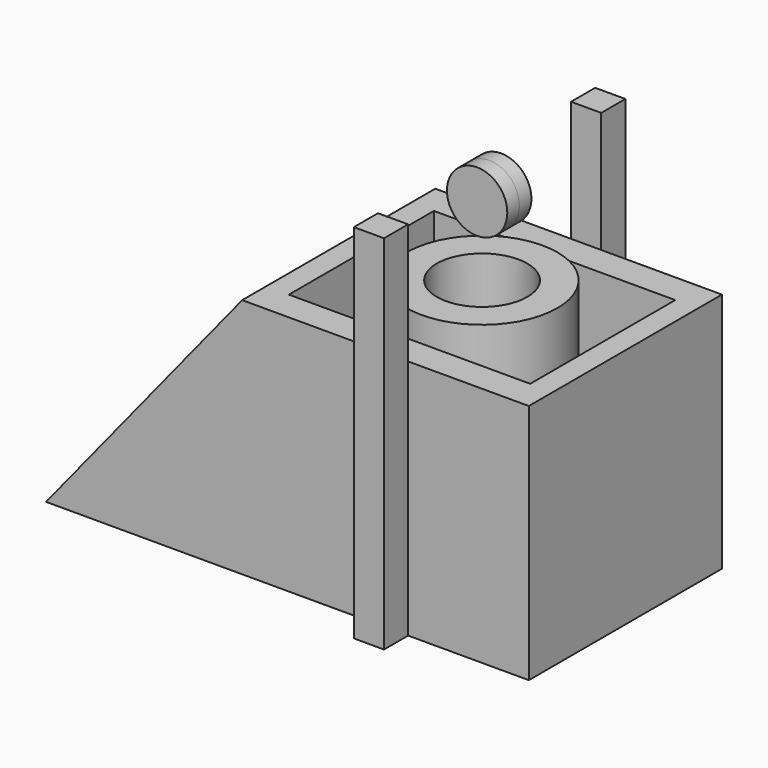
from build123d import *

# Parameters (mm, degrees)
F1_DEPTH  = 101.6
F2_W      = 101.6
F2_H      = 76.311862731
F3_DEPTH  = 95.25
F4_R      = 31.75
F5_DEPTH  = 101.6
F6_R      = 19.05
F7_DEPTH  = 159.004
F9_W      = 12.7
F9_H      = 50.8
F9_H_2    = 101.6
F10_DEPTH = 12.7
F12_DEPTH = 12.7
F17_R     = 12.7
F18_DEPTH = 6.35
F19_DEPTH = 6.35


# Not quite as in the source:
# - the program builds the solid bodies; features that only make, move or delete a surface that nothing else refers to are left out


with BuildPart() as f1:
    # F0 (on Front) → F1 (new body)
    with BuildSketch(Plane.XZ):
        Polygon((82.55, 101.6), (0, 0), (203.2, 0), (203.2, 101.6), align=None)
    extrude(amount=-F1_DEPTH)

    # F2 (on face) → F3 (cut)
    with BuildSketch(Plane.XY.offset(101.6)):
        with Locations((142.875, 50.8)):
            Rectangle(F2_W, F2_H)
    extrude(amount=-F3_DEPTH, mode=Mode.SUBTRACT)

    # F4 (on face) → F5 (join)
    with BuildSketch(Plane.XY.offset(6.35)):
        with Locations((142.875, 50.8)):
            Circle(F4_R)
    extrude(amount=F5_DEPTH)

    # F6 (on face) → F7 (cut)
    with BuildSketch(Plane.XY.offset(107.95)):
        with Locations((142.875, 50.8)):
            Circle(F6_R)
    extrude(amount=-F7_DEPTH, mode=Mode.SUBTRACT)

    # F9 (on face) → F10 (join)
    with BuildSketch(Plane(origin=(0, 101.6, 0), x_dir=(-1, 0, 0), z_dir=(0, 1, 0))):
        with Locations((-146.05, 127)):
            Rectangle(F9_W, F9_H)
        with Locations((-146.05, 50.8)):
            Rectangle(F9_W, F9_H_2)
    extrude(amount=F10_DEPTH)

    # F11 (on face) → F12 (join)
    with BuildSketch(Plane.XZ):
        Polygon((139.7, 0), (152.4, 0), (152.4, 101.6), (152.4, 152.4), (139.7, 152.4), (139.7, 101.6), align=None)
    extrude(amount=F12_DEPTH)


with BuildPart() as f18:
    # F17 (on offset) → F18 (new body)
    with BuildSketch(Plane.XZ.offset(-50.8)):
        with Locations((145.8720415831, 140.6437456608)):
            Circle(F17_R)
    extrude(amount=-F18_DEPTH)

    # F19 (add): a face of the model
    f19_faces = [f18.faces().sort_by_distance(p)[0] for p in [
        (145.8720415831, 50.8, 140.6437456608),
    ]]
    extrude(f19_faces, amount=F19_DEPTH)


solid = Compound([f1.part, f18.part])
